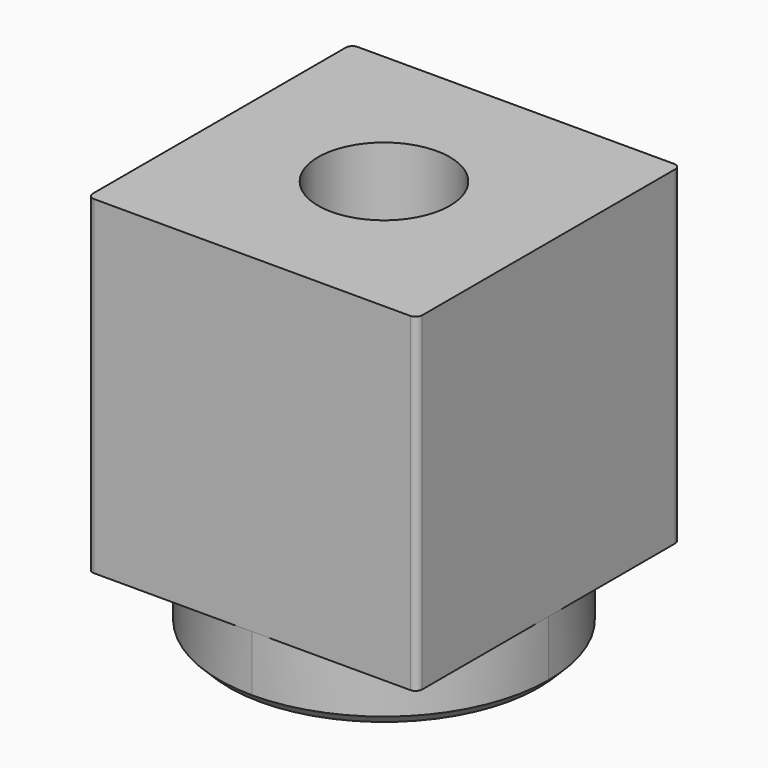
from build123d import *

# Parameters (mm, degrees)
F0_R     = 2
F1_DEPTH = 10
F2_DEPTH = 2
F4_R     = 0.2


# Not quite as in the source:
# - a fillet or chamfer that OpenCascade refuses, or shapes differently, is made with other operations: its cross-section is extruded or revolved along the edge and cut away or added


with BuildPart() as f1:
    # F0 (on Top) → F1 (new body)
    with BuildSketch(Plane.XY):
        with BuildLine():
            Line((5, 0), (5, 5))
            Line((5, 5), (0, 5))
            ThreePointArc((0, 5), (3.5355339059, 3.5355339059), (5, 0))
        make_face()
        with BuildLine():
            ThreePointArc((-5, 0), (-3.5355339059, 3.5355339059), (0, 5))
            Line((0, 5), (-5, 5))
            Line((-5, 5), (-5, 0))
        make_face()
        with BuildLine():
            ThreePointArc((5, 0), (3.5355339059, 3.5355339059), (0, 5))
            ThreePointArc((0, 5), (-3.5355339059, 3.5355339059), (-5, 0))
            ThreePointArc((-5, 0), (-3.5355339059, -3.5355339059), (0, -5))
            ThreePointArc((0, -5), (3.5355339059, -3.5355339059), (5, 0))
        make_face()
        Circle(F0_R, mode=Mode.SUBTRACT)
        with BuildLine():
            Line((5, -5), (5, 0))
            ThreePointArc((5, 0), (3.5355339059, -3.5355339059), (0, -5))
            Line((0, -5), (5, -5))
        make_face()
        with BuildLine():
            ThreePointArc((0, -5), (-3.5355339059, -3.5355339059), (-5, 0))
            Line((-5, 0), (-5, -5))
            Line((-5, -5), (0, -5))
        make_face()
    extrude(amount=F1_DEPTH)

    # F0 (on Top) → F2 (join)
    with BuildSketch(Plane.XY):
        with BuildLine():
            ThreePointArc((5, 0), (3.5355339059, 3.5355339059), (0, 5))
            ThreePointArc((0, 5), (-3.5355339059, 3.5355339059), (-5, 0))
            ThreePointArc((-5, 0), (-3.5355339059, -3.5355339059), (0, -5))
            ThreePointArc((0, -5), (3.5355339059, -3.5355339059), (5, 0))
        make_face()
        Circle(F0_R, mode=Mode.SUBTRACT)
    extrude(amount=-F2_DEPTH)

    # F3: chamfer of 0.3 on 1 edges, made by hand

    # F3_s1 → F3_t2 (revolve, cut)
    with BuildSketch(Plane.XZ):
        Polygon((-4.7, -2), (-5, -1.7), (-5, -2), align=None)
    revolve(axis=Axis((0, 0, -2), (0, 0, 1)), mode=Mode.SUBTRACT)

    # F4
    f4_edges = [f1.edges().sort_by_distance(p)[0] for p in [
        (5, 5, 5),
        (5, -5, 5),
        (-5, 5, 5),
        (-5, -5, 5),
    ]]
    fillet(f4_edges, radius=F4_R)


solid = f1.part
